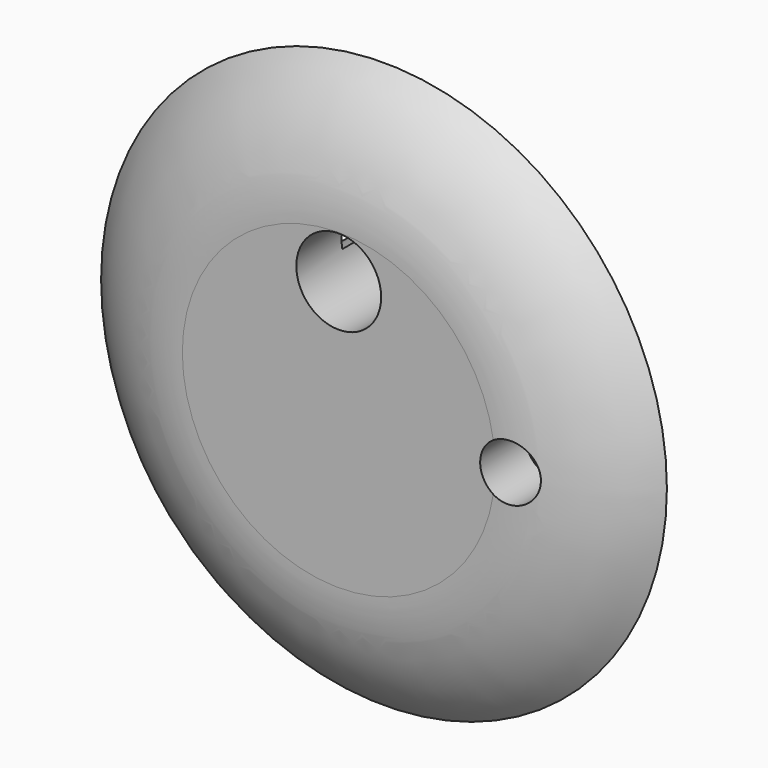
from build123d import *

# Parameters (mm, degrees)
F0_R     = 50
F1_DEPTH = 10
F2_R     = 20
F3_DEPTH = 25
F5_R     = 5
F6_DEPTH = 85.6401380152
F7_R     = 7.5
F8_DEPTH = 57.2151485831


# Not quite as in the source:
# - a fillet or chamfer that OpenCascade refuses, or shapes differently, is made with other operations: its cross-section is extruded or revolved along the edge and cut away or added


with BuildPart() as f1:
    # F0 (on Front) → F1 (new body)
    with BuildSketch(Plane.XZ):
        Circle(F0_R)
    extrude(amount=F1_DEPTH)

    # F2 (on face) → F3 (join)
    with BuildSketch(Plane(origin=(0, 0, 0), x_dir=(-1, 0, 0), z_dir=(0, 1, 0))):
        Circle(F2_R)
    extrude(amount=F3_DEPTH)

    # F5 (on offset) → F6 (cut)
    with BuildSketch(Plane.XZ.offset(10)):
        with Locations((30, 0)):
            Circle(F5_R)
    extrude(amount=-F6_DEPTH, mode=Mode.SUBTRACT)

    # F7 (on face) → F8 (cut)
    with BuildSketch(Plane.XZ.offset(10)):
        with Locations((0, 20)):
            Circle(F7_R)
    extrude(amount=-F8_DEPTH, mode=Mode.SUBTRACT)

    # F9: fillet of radius 29.9906943199 on 1 edges, made by hand

    # F9_s1 → F9_t2 (revolve, cut)
    with BuildSketch(Plane.XY):
        with BuildLine():
            ThreePointArc((50, 0), (39.8890312916, -7.3860891689), (27.643482239, -10))
            Line((27.643482239, -10), (50, -10))
            Line((50, -10), (50, 0))
        make_face()
    revolve(axis=Axis((0, -10, 0), (0, -1, 0)), mode=Mode.SUBTRACT)


solid = f1.part
